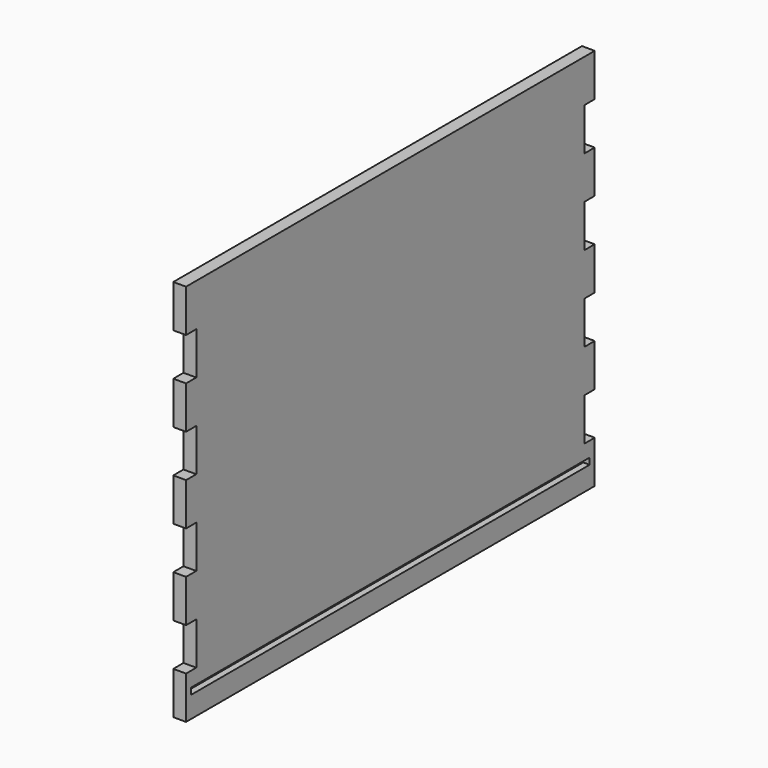
from build123d import *

# Parameters (mm, degrees)
F0_W     = 6
F0_H     = 240
F1_DEPTH = 180
F3_START = -3
F2_W     = 3
F2_H     = 3
F3_DEPTH = 234
F4_W     = 6
F4_H     = 20
F5_DEPTH = 6.001


with BuildPart() as f1:
    # F0 (on Top) → F1 (new body)
    with BuildSketch(Plane.XY):
        Rectangle(F0_W, F0_H)
    extrude(amount=F1_DEPTH)

    # F2 (on face) → F3 (cut)
    with BuildSketch(Plane.XZ.offset(120).offset(F3_START)):
        with Locations((1.5, 11.5)):
            Rectangle(F2_W, F2_H)
    extrude(amount=-F3_DEPTH, mode=Mode.SUBTRACT)

    # F4 (on face) → F5 (cut, through all)
    with BuildSketch(Plane.YZ.offset(3)):
        with Locations((-117, 30)):
            Rectangle(F4_W, F4_H)
        with Locations((-117, 70)):
            Rectangle(F4_W, F4_H)
        with Locations((-117, 110)):
            Rectangle(F4_W, F4_H)
        with Locations((-117, 150)):
            Rectangle(F4_W, F4_H)
        with Locations((117, 150)):
            Rectangle(F4_W, F4_H)
        with Locations((117, 110)):
            Rectangle(F4_W, F4_H)
        with Locations((117, 70)):
            Rectangle(F4_W, F4_H)
        with Locations((117, 30)):
            Rectangle(F4_W, F4_H)
    extrude(amount=-F5_DEPTH, mode=Mode.SUBTRACT)


solid = f1.part
